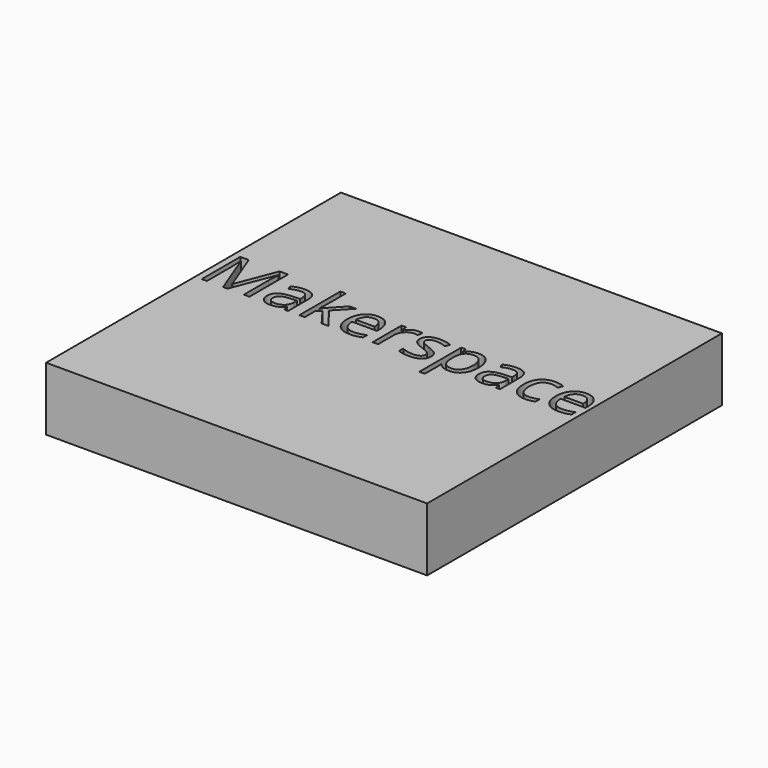
from build123d import *

# Parameters (mm, degrees)
F0_W         = 152.6714786887
F0_H         = 147.6293727756
F1_DEPTH     = 25.4
F2_TEXT_SIZE = 27.0274801839
F3_DEPTH     = 12.7


# Not quite as in the source:
# - Text() gives the source's letters only with a copy of the font that has no kerning and outlines rounded to 1/6400 em; it was checked with that copy


with BuildPart() as f1:
    # F0 (on Top) → F1 (new body)
    with BuildSketch(Plane.XY):
        with Locations((0.0298656523, -0.4975534976)):
            Rectangle(F0_W, F0_H)
    extrude(amount=F1_DEPTH)

    # F2 (on face) → F3 (cut)
    with BuildSketch(Plane.XY.offset(25.4)):
        with Locations((-76.305873692, 0.3410191424)):
            Text('Makerspace', F2_TEXT_SIZE, font='Open Sans', text_align=(TextAlign.LEFT, TextAlign.BOTTOM))
    extrude(amount=-F3_DEPTH, mode=Mode.SUBTRACT)


solid = f1.part
